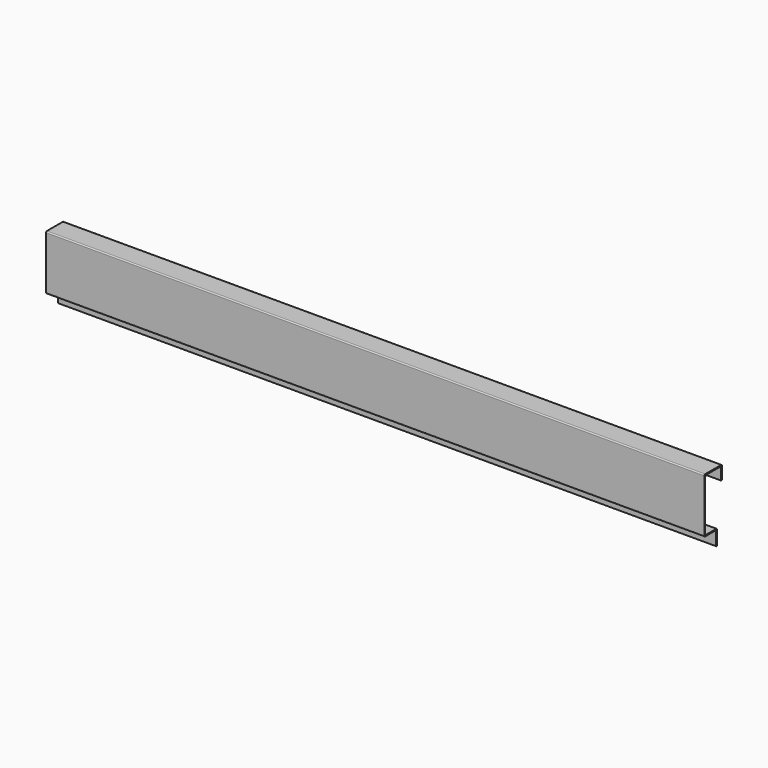
from build123d import *

# Parameters (mm, degrees)
F1_DEPTH = 1200
F2_R     = 2


# Not quite as in the source:
# - a feature names something its author has since deleted; it is built from what else it names


with BuildPart() as f1:
    # F0 (on Right) → F1 (new body)
    with BuildSketch(Plane.YZ):
        Polygon((-18.8378913403, 177.8021101952), (-18.8378913403, 154.8021101952), (-16.8378913403, 154.8021101952), (-16.8378913403, 179.8021101952), (-56.8378913403, 179.8021101952), (-56.8378913403, 79.8021101952), (-29.8378913403, 79.8021101952), (-29.8378913403, 53.8021101952), (-27.8378913403, 53.8021101952), (-27.8378913403, 81.8021101952), (-54.8378913403, 81.8021101952), (-54.8378913403, 177.8021101952), align=None)
    extrude(amount=F1_DEPTH)

    # F2
    f2_edges = [f1.edges().sort_by_distance(p)[0] for p in [
        (600, -56.837891, 179.80211),
        (600, -16.837891, 179.80211),
        (600, -56.837891, 79.80211),
        (600, -27.837891, 81.80211),
        (600, -54.837891, 81.80211),
        (600, -29.837891, 79.80211),
        (600, -18.837891, 177.80211),
        (600, -54.837891, 177.80211),
    ]]
    fillet(f2_edges, radius=F2_R)


solid = f1.part
